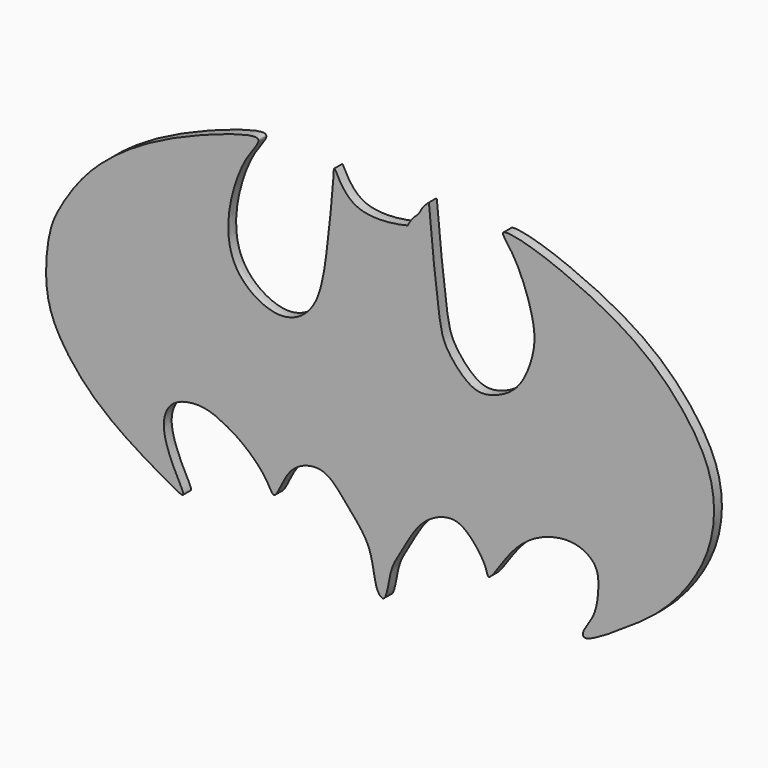
from build123d import *

# Parameters (mm, degrees)
F1_DEPTH = 0.8


with BuildPart() as f1:
    # F0 (on Front) → F1 (new body)
    with BuildSketch(Plane.XZ):
        with BuildLine():
            add(Edge.make_bspline(
                [(-30.6339133531, 47.4556051195), (-29.1970439347, 46.7424352018), (-26.4241559146, 47.3977409327), (-26.433064808, 47.4515625121), (-26.0364247334, 48.1623017065), (-25.5310986829, 48.4761313494), (-25.2985992431, 49.062598106), (-24.8916319437, 49.4713739526), (-24.6956028438, 49.6661258771), (-24.6933820037, 49.1791627185), (-24.5212597199, 47.6573624), (-24.3528822518, 45.7176482219), (-23.9423982587, 42.2457508459), (-23.7693975554, 41.1275380273), (-23.4791907397, 39.8314321598), (-22.235135181, 38.2188072736), (-20.8344879816, 37.2178013789), (-19.2761031551, 37.4679405039), (-17.2750622898, 38.5432967534), (-16.1199944645, 41.3827039732), (-15.9842211236, 43.8539897344), (-17.5486770033, 48.0568183611), (-19.120205725, 49.6237354908), (-17.2319165362, 49.4546607679), (-13.458660532, 48.1713081468), (-7.8538258402, 45.4449957959), (-3.7902562732, 41.5601630058), (-1.146100923, 37.057445338), (-1.5862458756, 31.4849338292), (-5.2117922666, 26.6794432944), (-8.4220807457, 24.477316607), (-12.0315061194, 22.139725368), (-12.2660175457, 22.9558323762), (-11.1137534422, 24.265383152), (-10.8480420344, 26.3296599667), (-10.9083270571, 28.1094802065), (-12.8406604283, 29.34196278), (-15.9445604089, 28.6916529007), (-18.1922573663, 26.7625175489), (-19.9002290851, 23.8104961322), (-20.0108370977, 25.1361271322), (-21.4422605897, 27.0374090029), (-22.9363826988, 27.8066167594), (-25.4682369528, 26.7177390833), (-26.8903998407, 23.8679244709), (-27.9338840392, 22.4267495747), (-28.1557237299, 19.6143213392), (-29.1676796491, 20.4519737133), (-29.2603411858, 23.3481975888), (-31.0381527399, 25.2962250498), (-32.5943375574, 27.2795247026), (-34.0218230383, 27.8123166401), (-36.3097752602, 27.0278564541), (-37.2592867012, 23.8497674532), (-37.8859439307, 25.5642559362), (-39.8214038536, 27.4914896447), (-41.7435130772, 28.5271939738), (-43.1892772307, 29.0969234057), (-45.7001941749, 28.8172135101), (-46.771704854, 26.4803427995), (-45.3092938904, 23.3609791947), (-44.4190878483, 21.7871922004), (-46.0944781579, 22.7072220824), (-48.6273486636, 24.1617147749), (-51.7835662194, 26.3454689678), (-54.3085503485, 29.1491064407), (-56.1934192158, 32.5998967268), (-55.7987483092, 37.3534782718), (-54.9640418668, 39.300897697), (-53.0266786935, 42.376485024), (-49.7827044639, 45.2758012105), (-45.0554770101, 47.9482415519), (-38.5263946137, 50.1609622969), (-38.6172948871, 49.2622622602), (-39.6802125897, 48.1045147813), (-41.1961642708, 44.3840462261), (-41.1840608453, 39.502660473), (-36.9375796447, 36.9007174027), (-33.6976927333, 38.8202653699), (-32.9937036356, 43.4290674848), (-32.4852932523, 48.6538676759), (-32.459910459, 50.1118633066), (-31.7995056205, 48.0341304404), (-30.6339133531, 47.4556051195)],
                knots=[0, 0, 0, 0, 0.0164897023, 0.0181932161, 0.0250875305, 0.0315744864, 0.0378667573, 0.0441068391, 0.0473232532, 0.0518199658, 0.0616835418, 0.0735401849, 0.0884960115, 0.0971382019, 0.1061090071, 0.1176340634, 0.1279299114, 0.1376090436, 0.1495036899, 0.1631580436, 0.1760579293, 0.1933918116, 0.2031418477, 0.2114875312, 0.2278855455, 0.2482028363, 0.2673203738, 0.2852978665, 0.3038363463, 0.3231204479, 0.340139792, 0.3554271922, 0.3601284442, 0.3704507986, 0.3822597705, 0.3925513517, 0.4037955933, 0.4176272918, 0.4323334345, 0.4451959796, 0.4516420372, 0.4642075212, 0.4742755862, 0.4869136622, 0.5010711364, 0.5125771326, 0.524473355, 0.530756097, 0.5442580137, 0.5575952666, 0.5701702912, 0.5796055392, 0.5918224846, 0.6043237973, 0.6122046447, 0.6259464538, 0.6378567684, 0.647860017, 0.6599070354, 0.671751017, 0.6870189335, 0.6954851353, 0.704171588, 0.7185088804, 0.7343627771, 0.7499338996, 0.7658898387, 0.7830141311, 0.7948294928, 0.8097882046, 0.8263790449, 0.8465404079, 0.8661544712, 0.8706844925, 0.8803887688, 0.896623927, 0.9139622054, 0.9303122575, 0.9442198153, 0.961819933, 0.9806816595, 0.98662351, 1, 1, 1, 1], degree=3))
        make_face()
    extrude(amount=F1_DEPTH)


solid = f1.part
